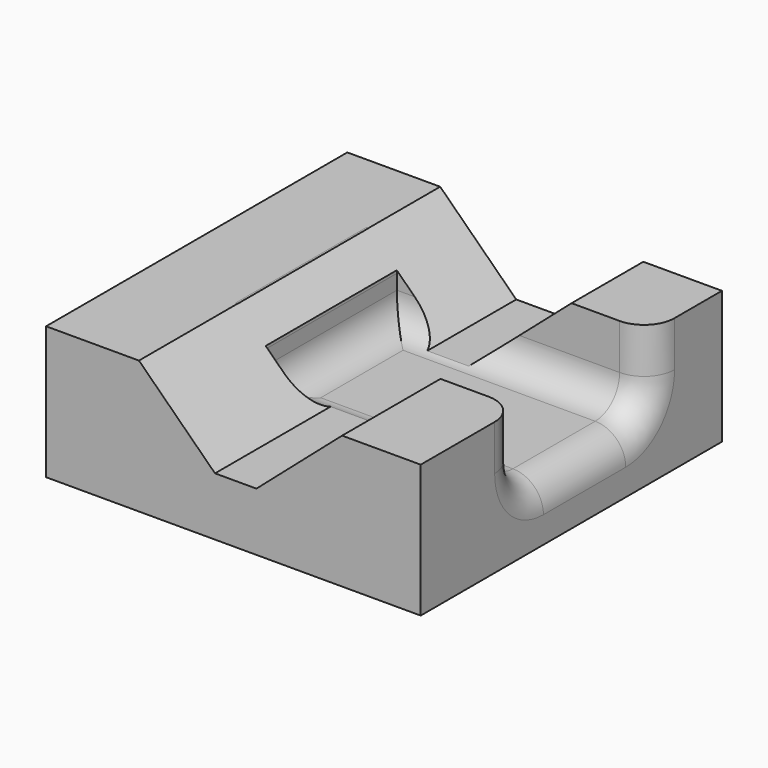
from build123d import *

# Parameters (mm, degrees)
F0_W     = 93.5896597803
F0_H     = 94.0682813525
F1_DEPTH = 33.197
F2_W     = 63.2629562169
F2_H     = 40.9446330741
F3_DEPTH = 18.96077
F4_F1_R  = 7.62
F4_F2_R  = 7.62
F6_DEPTH = 123.1075


with BuildPart() as f1:
    # F0 (on Top) → F1 (new body)
    with BuildSketch(Plane.XY):
        with Locations((-5.7506207377, 2.1532103419)):
            Rectangle(F0_W, F0_H)
    extrude(amount=-F1_DEPTH)

    # F2 (on face) → F3 (cut)
    with BuildSketch(Plane.XY):
        with Locations((9.412731044, 6.3009518199)):
            Rectangle(F2_W, F2_H)
    extrude(amount=-F3_DEPTH, mode=Mode.SUBTRACT)

    # F4: fillet of radius 7.62 on 5 edges, made by hand

    # F4_f1
    f4_f1_edges = [f1.edges().sort_by_distance(p)[0] for p in [
        (9.412731044, -14.1713647172, -18.96077),
        (9.412731044, 26.7732683569, -18.96077),
        (-22.2187470645, 6.3009518199, -18.96077),
    ]]
    fillet(f4_f1_edges, radius=F4_F1_R)

    # F4_f2
    f4_f2_edges = [f1.edges().sort_by_distance(p)[0] for p in [
        (41.0442091525, 6.3009518199, -18.96077),
        (-22.2187470645, 6.3009518199, 0),
        (41.0442091525, -11.9395183898, -16.7289236726),
        (41.0442091525, 24.5414220296, -16.7289236726),
    ]]
    fillet(f4_f2_edges, radius=F4_F2_R)

    # F5 (on face) → F6 (cut)
    with BuildSketch(Plane(origin=(0, 49.1873510182, 0), x_dir=(-1, 0, 0), z_dir=(0, 1, 0))):
        Polygon((29.3431449682, 0), (-21.4069634676, 0), (0, -18.6201948673), (10.3417439386, -18.6201948673), align=None)
    extrude(amount=-F6_DEPTH, mode=Mode.SUBTRACT)


solid = f1.part
